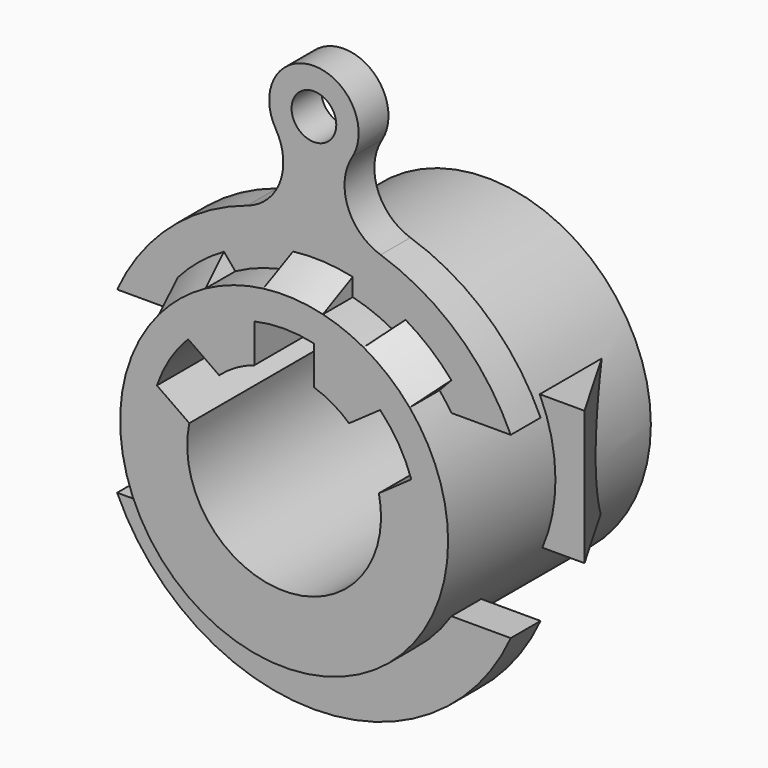
from build123d import *

# Parameters (mm, degrees)
F0_R         = 44
F1_DEPTH     = 68
F3_R         = 6
F4_DEPTH     = 10
F7_DEPTH     = 10
F8_T4_ANGLE  = 83.7942350081
F8_T9_ANGLE  = 83.7884226617
F8_T14_ANGLE = 83.7665747307
F11_DEPTH    = 25
F12_T4_DEPTH = 165.3542877323
F12_S5_R     = 44
F12_T6_DEPTH = 86
F13_T4_DEPTH = 165.3542877323
F13_S5_R     = 44
F13_T6_DEPTH = 85


# Not quite as in the source:
# - a fillet or chamfer that OpenCascade refuses, or shapes differently, is made with other operations: its cross-section is extruded or revolved along the edge and cut away or added


with BuildPart() as f1:
    # F0 (on Front) → F1 (new body)
    with BuildSketch(Plane.XZ):
        Circle(F0_R)
        with BuildLine():
            ThreePointArc((-17.4170906965, 19.3040138746), (-12.9958030986, 22.5190830591), (-8, 24.7386337537))
            Line((-8, 24.7386337537), (-8, 35.0998575496))
            ThreePointArc((-8, 35.0998575496), (0, 36), (8, 35.0998575496))
            Line((8, 35.0998575496), (8, 24.7386337537))
            ThreePointArc((8, 24.7386337537), (12.9958030986, 22.5190830591), (17.4170906965, 19.3040138746))
            Line((17.4170906965, 19.3040138746), (25.7612918983, 25.1466864563))
            ThreePointArc((25.7612918983, 25.1466864563), (30.7135727536, 18.7796818053), (34.1239224392, 11.4698699802))
            Line((34.1239224392, 11.4698699802), (25.4359194285, 5.3864647801))
            ThreePointArc((25.4359194285, 5.3864647801), (0, -26), (-25.4359194285, 5.3864647801))
            Line((-25.4359194285, 5.3864647801), (-34.1239224392, 11.4698699802))
            ThreePointArc((-34.1239224392, 11.4698699802), (-30.7135727536, 18.7796818053), (-25.7612918983, 25.1466864563))
            Line((-25.7612918983, 25.1466864563), (-17.4170906965, 19.3040138746))
        make_face(mode=Mode.SUBTRACT)
    extrude(amount=F1_DEPTH)

    # F3 (on offset) → F4 (join)
    with BuildSketch(Plane.XZ.offset(48)):
        with BuildLine():
            ThreePointArc((-10.252187236, 75.7636022514), (-9.0876412514, 63.6171726174), (-17.8938638331, 55.1707317073))
            ThreePointArc((-17.8938638331, 55.1707317073), (-38.6311115614, 43.2624227191), (-52.8015151298, 24))
            Line((-52.8015151298, 24), (-36.8781778292, 24))
            ThreePointArc((-36.8781778292, 24), (0, 44), (36.8781778292, 24))
            Line((36.8781778292, 24), (52.8015151298, 24))
            ThreePointArc((52.8015151298, 24), (38.6311115614, 43.2624227191), (17.8938638331, 55.1707317073))
            ThreePointArc((17.8938638331, 55.1707317073), (9.0876412514, 63.6171726174), (10.252187236, 75.7636022514))
            ThreePointArc((10.252187236, 75.7636022514), (0, 94), (-10.252187236, 75.7636022514))
        make_face()
        with Locations((0, 82)):
            Circle(F3_R, mode=Mode.SUBTRACT)
        with BuildLine():
            ThreePointArc((36.8781778292, -24), (0, -44), (-36.8781778292, -24))
            Line((-36.8781778292, -24), (-52.8015151298, -24))
            ThreePointArc((-52.8015151298, -24), (0, -58), (52.8015151298, -24))
            Line((52.8015151298, -24), (36.8781778292, -24))
        make_face()
    extrude(amount=F4_DEPTH)

    # F6 (on offset) → F7 (join)
    with BuildSketch(Plane.XZ.offset(58)):
        with BuildLine():
            Line((-36.7577330787, 32.4016829643), (-33.5029734135, 28.5228114402))
            ThreePointArc((-33.5029734135, 28.5228114402), (-27.7578301996, 34.1394619555), (-21.0871377876, 38.6177759578))
            Line((-21.0871377876, 38.6177759578), (-24.3586089556, 42.5165634753))
            ThreePointArc((-24.3586089556, 42.5165634753), (-30.9738521636, 37.9686776455), (-36.7577330787, 32.4016829643))
        make_face()
        with BuildLine():
            ThreePointArc((-5.5873169023, 43.6438070043), (2.4537097938, 43.9315297736), (10.4126830977, 42.7501582536))
            Line((10.4126830977, 42.7501582536), (10.4126830977, 47.8808524434))
            ThreePointArc((10.4126830977, 47.8808524434), (2.4455798994, 48.9389327525), (-5.5873169023, 48.6804056046))
            Line((-5.5873169023, 48.6804056046), (-5.5873169023, 43.6438070043))
        make_face()
        with BuildLine():
            Line((33.6836647587, 28.3091986539), (37.1178360984, 31.9885329982))
            ThreePointArc((37.1178360984, 31.9885329982), (31.3875014297, 37.6274468175), (24.8122261451, 42.2534428624))
            Line((24.8122261451, 42.2534428624), (21.306338137, 38.4972720487))
            ThreePointArc((21.306338137, 38.4972720487), (27.9629096213, 33.9716894709), (33.6836647587, 28.3091986539))
        make_face()
    extrude(amount=F7_DEPTH)

    # F8: chamfer of 5 x 10.7225346025 on 3 edges, made by hand


with BuildPart() as f8_tool2:
    # F8_s3 → F8_t4 (revolve)
    with BuildSketch(Plane(origin=(0, 0, 0), x_dir=(0, 1, 0), z_dir=(0.1438242317, 0, -0.989603249))):
        Polygon((-68, 44), (-57.2774653975, 49), (-68, 49), align=None)
    revolve(axis=Axis((0, -68, 0), (0, -1, 0)), revolution_arc=F8_T4_ANGLE)

    split(bisect_by=Plane.XZ.offset(58), keep=Keep.TOP)


with BuildPart() as f1_1:
    add(f1.part)

    # F8_t1: cut F8_tool2
    add(f8_tool2.part, mode=Mode.SUBTRACT)


with BuildPart() as f8_tool7:
    # F8_s8 → F8_t9 (revolve)
    with BuildSketch(Plane(origin=(0, 0, 0), x_dir=(0, 1, 0), z_dir=(0.7101236851, 0, -0.7040769502))):
        Polygon((-68, 44), (-57.2774653975, 49), (-68, 49), align=None)
    revolve(axis=Axis((0, -68, 0), (0, -1, 0)), revolution_arc=F8_T9_ANGLE)

    split(bisect_by=Plane.XZ.offset(58), keep=Keep.TOP)


with BuildPart() as f1_2:
    add(f1_1.part)

    # F8_t6: cut F8_tool7
    add(f8_tool7.part, mode=Mode.SUBTRACT)


with BuildPart() as f8_tool12:
    # F8_s13 → F8_t14 (revolve)
    with BuildSketch(Plane(origin=(0, 0, 0), x_dir=(0, 1, 0), z_dir=(0.9989090113, 0, -0.0466988996))):
        Polygon((-68, 44), (-57.2774653975, 49), (-68, 49), align=None)
    revolve(axis=Axis((0, -68, 0), (0, -1, 0)), revolution_arc=F8_T14_ANGLE)

    split(bisect_by=Plane.XZ.offset(58), keep=Keep.TOP)


with BuildPart() as f1_3:
    add(f1_2.part)

    # F8_t11: cut F8_tool12
    add(f8_tool12.part, mode=Mode.SUBTRACT)

    # F10 (on offset) → F11 (join)
    with BuildSketch(Plane.XZ.offset(32)):
        with BuildLine():
            ThreePointArc((39.7816943244, 18.7993828803), (42.9324734337, 9.6334170917), (44, 0))
            ThreePointArc((44, 0), (43.1157719293, -8.7766856466), (40.4986267755, -17.2006171197))
            Line((40.4986267755, -17.2006171197), (51.7816943244, -17.2006171197))
            Line((51.7816943244, -17.2006171197), (51.7816943244, 18.7993828803))
            Line((51.7816943244, 18.7993828803), (39.7816943244, 18.7993828803))
        make_face()
        with BuildLine():
            ThreePointArc((-40.4986267755, -17.2006171197), (-43.9912774192, 0.8760770652), (-39.7816943244, 18.7993828803))
            Line((-39.7816943244, 18.7993828803), (-51.7816943244, 18.7993828803))
            Line((-51.7816943244, 18.7993828803), (-51.7816943244, -17.2006171197))
            Line((-51.7816943244, -17.2006171197), (-40.4986267755, -17.2006171197))
        make_face()
    extrude(amount=-F11_DEPTH)

    # F12: chamfer of 25 x 14.4337567297 on 1 edges, made by hand


with BuildPart() as f12_tool2:
    # F12_s3 → F12_t4 (new body)
    with BuildSketch(Plane.XY.offset(-81.8777609858)):
        with BuildLine():
            Line((36.8479375946, -6.1339745962), (52.2816943244, -32.8660254038))
            Line((52.2816943244, -32.8660254038), (52.7816943244, -32.8660254038))
            ThreePointArc((52.7816943244, -32.8660254038), (52.2816943244, -19.9330127019), (52.2816943244, -7))
            Line((52.2816943244, -7), (51.7816943244, -6.5))
            ThreePointArc((51.7816943244, -6.5), (44.3148159595, -6.5), (36.8479375946, -5.6339745962))
            Line((36.8479375946, -5.6339745962), (36.8479375946, -6.1339745962))
        make_face()
    extrude(amount=F12_T4_DEPTH)

    # F12_s5 → F12_t6 (cut, symmetric)
    with BuildSketch(Plane.XZ.offset(19.3)):
        Circle(F12_S5_R)
    extrude(amount=F12_T6_DEPTH, both=True, mode=Mode.SUBTRACT)


with BuildPart() as f1_4:
    add(f1_3.part)

    # F12_t1: cut F12_tool2
    add(f12_tool2.part, mode=Mode.SUBTRACT)

    # F13: chamfer of 25 x 14.4337567297 on 1 edges, made by hand


with BuildPart() as f13_tool2:
    # F13_s3 → F13_t4 (new body)
    with BuildSketch(Plane.XY.offset(83.4765267465)):
        Polygon((-37.3479375946, -7), (-51.7816943244, -32), (-51.7816943244, -7), align=None)
    extrude(amount=-F13_T4_DEPTH)

    # F13_s5 → F13_t6 (cut, symmetric)
    with BuildSketch(Plane.XZ.offset(19.5)):
        Circle(F13_S5_R)
    extrude(amount=F13_T6_DEPTH, both=True, mode=Mode.SUBTRACT)


with BuildPart() as f1_5:
    add(f1_4.part)

    # F13_t1: cut F13_tool2
    add(f13_tool2.part, mode=Mode.SUBTRACT)


solid = f1_5.part
